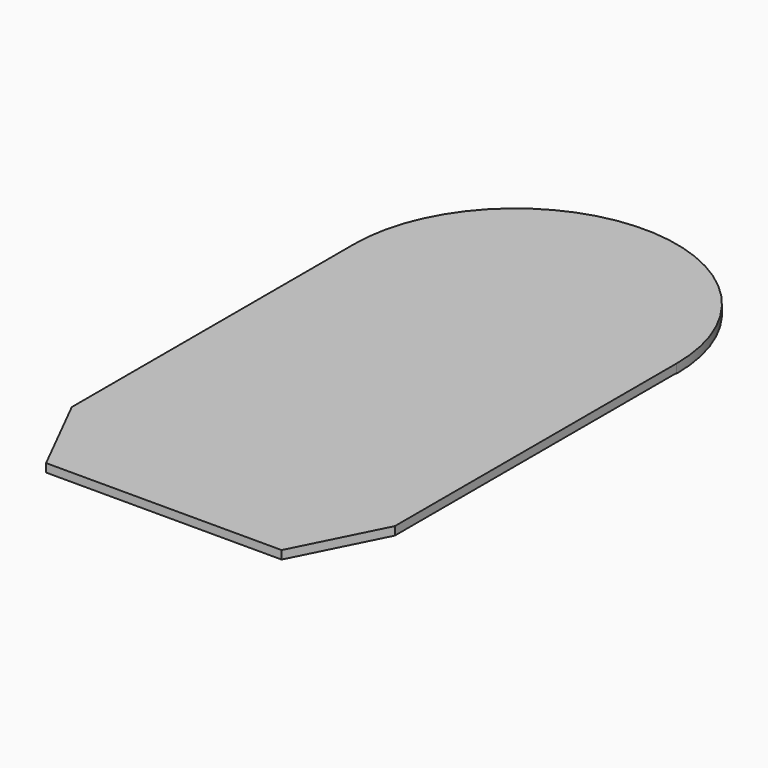
from build123d import *

# Parameters (mm, degrees)
F0_W     = 109.6518
F0_H     = 149.225
F1_DEPTH = 2.8448
F3_DEPTH = 25.4
F5_DEPTH = 3.048
F9_DEPTH = 107.442


# Not quite as in the source:
# - a feature names something its author has since deleted; it is built from what else it names


with BuildPart() as f1:
    # F0 (on Top) → F1 (new body)
    with BuildSketch(Plane.XY):
        with Locations((13.2645608256, 0)):
            Rectangle(F0_W, F0_H)
    extrude(amount=F1_DEPTH)

    # F2 (on face) → F3 (cut)
    with BuildSketch(Plane.XY.offset(2.8448)):
        Polygon((68.0904608256, -74.6125), (27.7860667557, -74.6125), (68.0904608256, -75.2405971289), align=None)
        Polygon((-41.5613391744, -75.712069869), (-25.0190570951, -74.6125), (-41.5613391744, -74.6125), align=None)
    extrude(amount=-F3_DEPTH, mode=Mode.SUBTRACT)

    # F4 (on face) → F5 (join)
    with BuildSketch(Plane.XY.offset(2.8448)):
        with BuildLine():
            Line((-41.5613391744, 74.6125), (68.0904608256, 74.6125))
            ThreePointArc((68.0904608256, 74.6125), (13.2645608256, 129.4384), (-41.5613391744, 74.6125))
        make_face()
    extrude(amount=-F5_DEPTH)


with BuildPart() as f1_1:
    # F6: moved
    add(f1.part.moved(Location((-10.668, 0, 0))))


with BuildPart() as f1_2:
    # F7: moved
    add(f1_1.part.moved(Location((-2.794, 0, 0))))

    # F8 (on Top) → F9 (cut)
    with BuildSketch(Plane.XY):
        Polygon((-55.1044642925, -45.067888195), (-55.1044642925, -74.785888195), (-40.1565642925, -74.785888195), align=None)
        Polygon((54.6766667015, -45.0012958965), (39.7287667015, -74.7192958965), (54.6766667015, -74.7192958965), align=None)
    extrude(amount=F9_DEPTH, mode=Mode.SUBTRACT)


solid = f1_2.part
